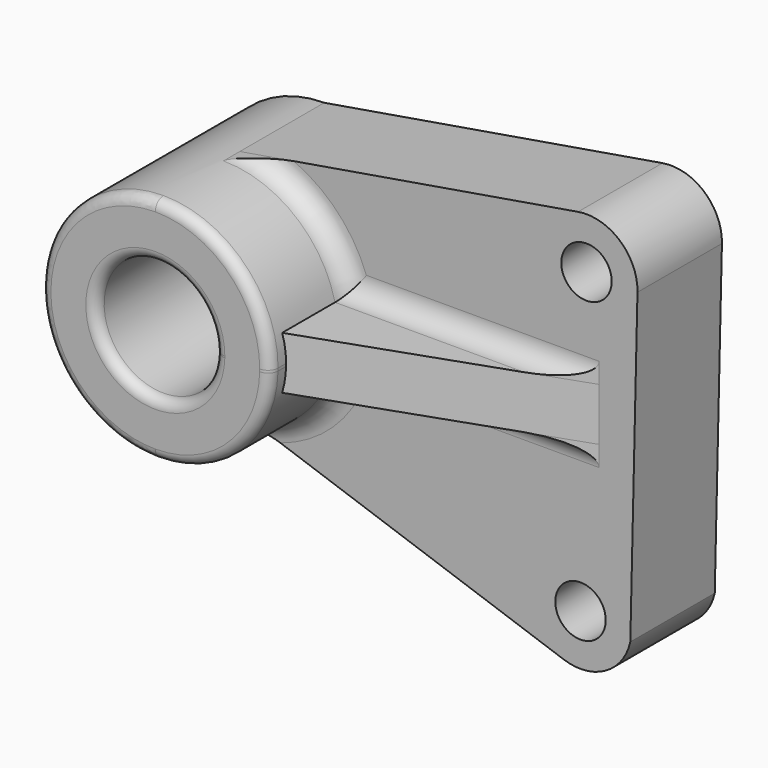
from build123d import *

# Parameters (mm, degrees)
F1_DEPTH     = 12.7
F2_DEPTH     = 25.4
F3_R         = 3.0339595682
F4_DEPTH     = 25.4
F5_R         = 1.2264204897
F7_DEPTH     = 3.175
F8_T4_ANGLE  = 97.0773840638
F8_T9_DEPTH  = 34.7132171162
F8_T14_ANGLE = 97.0773840638
F8_T19_DEPTH = 34.7132171162


# Not quite as in the source:
# - a fillet or chamfer that OpenCascade refuses, or shapes differently, is made with other operations: its cross-section is extruded or revolved along the edge and cut away or added


with BuildPart() as f1:
    # F0 (on Front) → F1 (new body)
    with BuildSketch(Plane.XZ):
        with BuildLine():
            ThreePointArc((0, -13.789825828), (9.6376295499, -9.8628288552), (13.7861481364, -0.3184586768))
            ThreePointArc((13.7861481364, -0.3184586768), (13.7889063745, -0.1592399559), (13.789825828, 0))
            ThreePointArc((13.789825828, 0), (9.7508793544, 9.7508793544), (0, 13.789825828))
            ThreePointArc((0, 13.789825828), (-13.789825828, 0), (0, -13.789825828))
        make_face()
        with BuildLine():
            ThreePointArc((7.1353728529, -0.1648264167), (-7.1368004494, 0.0824187037), (7.137276336, 0))
            ThreePointArc((7.137276336, 0), (7.1368004494, -0.0824187037), (7.1353728529, -0.1648264167))
        make_face(mode=Mode.SUBTRACT)
        with BuildLine():
            ThreePointArc((13.789825828, 0), (13.7889063745, -0.1592399559), (13.7861481364, -0.3184586768))
            ThreePointArc((13.7861481364, -0.3184586768), (9.6376295499, -9.8628288552), (0, -13.789825828))
            Line((0, -13.789825828), (38.9815755188, -27.3394305259))
            ThreePointArc((38.9815755188, -27.3394305259), (43.9885292005, -26.9000346666), (46.9867042389, -22.8659795937))
            Line((46.9867042389, -22.8659795937), (47.8485122544, 14.4418842975))
            ThreePointArc((47.8485122544, 14.4418842975), (45.7311207367, 19.22142423), (40.6978976177, 20.6335197794))
            Line((40.6978976177, 20.6335197794), (0, 13.789825828))
            ThreePointArc((0, 13.789825828), (9.7508793544, 9.7508793544), (13.789825828, 0))
        make_face()
    extrude(amount=F1_DEPTH)

    # F0 (on Front) → F2 (join)
    with BuildSketch(Plane.XZ):
        with BuildLine():
            ThreePointArc((0, -13.789825828), (9.6376295499, -9.8628288552), (13.7861481364, -0.3184586768))
            ThreePointArc((13.7861481364, -0.3184586768), (13.7889063745, -0.1592399559), (13.789825828, 0))
            ThreePointArc((13.789825828, 0), (9.7508793544, 9.7508793544), (0, 13.789825828))
            ThreePointArc((0, 13.789825828), (-13.789825828, 0), (0, -13.789825828))
        make_face()
        with BuildLine():
            ThreePointArc((7.1353728529, -0.1648264167), (-7.1368004494, 0.0824187037), (7.137276336, 0))
            ThreePointArc((7.137276336, 0), (7.1368004494, -0.0824187037), (7.1353728529, -0.1648264167))
        make_face(mode=Mode.SUBTRACT)
    extrude(amount=F2_DEPTH)

    # F3 (on face) → F4 (cut)
    with BuildSketch(Plane.XZ.offset(12.7)):
        with Locations((40.9957959094, -21.5446131849)):
            Circle(F3_R)
        with Locations((41.715248914, 14.5835620822)):
            Circle(F3_R)
    extrude(amount=-F4_DEPTH, mode=Mode.SUBTRACT)

    # F5
    f5_edges = [f1.edges().sort_by_distance(p)[0] for p in [
        (0, -25.4, 13.789826),
        (-7.137276, -25.4, 0),
    ]]
    fillet(f5_edges, radius=F5_R)

    # F6 (on Top) → F7 (join, symmetric)
    with BuildSketch(Plane.XY):
        Polygon((13.3344670758, -12.2673781589), (13.3344670758, -23.1246650219), (44.4674044847, -12.2673781589), align=None)
    extrude(amount=F7_DEPTH, both=True)

    # F8: fillet of radius 2.4528409794 on 4 edges, made by hand


with BuildPart() as f8_tool2:
    # F8_s3 → F8_t4 (revolve)
    with BuildSketch(Plane(origin=(0, 0, 0), x_dir=(0, 1, 0), z_dir=(0.0543746304, 0, 0.9985206055))):
        with BuildLine():
            ThreePointArc((-15.1528409794, -13.789825828), (-13.4184204897, -14.5082463177), (-12.7, -16.2426668074))
            Line((-12.7, -16.2426668074), (-12.6509431804, -16.2426668074))
            Line((-12.6509431804, -16.2426668074), (-12.6509431804, -13.7407690084))
            Line((-12.6509431804, -13.7407690084), (-15.1528409794, -13.7407690084))
            Line((-15.1528409794, -13.7407690084), (-15.1528409794, -13.789825828))
        make_face()
    revolve(axis=Axis((0, -12.7, 0), (0, 1, 0)), revolution_arc=F8_T4_ANGLE)

    split(bisect_by=Plane(origin=(-4.2765210661, 0, -12.3033499954), x_dir=(0, 1, 0), z_dir=(0.3283216608, 0, 0.9445659781)), keep=Keep.TOP)


with BuildPart() as f1_1:
    add(f1.part)

    # F8_t1: union F8_tool2
    add(f8_tool2.part)


with BuildPart() as f8_tool7:
    # F8_s8 → F8_t9 (new body)
    with BuildSketch(Plane.YZ.offset(45.6797155903)):
        with BuildLine():
            ThreePointArc((-12.7, -5.6278409794), (-13.4184204897, -3.8934204897), (-15.1528409794, -3.175))
            Line((-15.1528409794, -3.175), (-15.1528409794, -3.1259431804))
            Line((-15.1528409794, -3.1259431804), (-12.6509431804, -3.1259431804))
            Line((-12.6509431804, -3.1259431804), (-12.6509431804, -5.6278409794))
            Line((-12.6509431804, -5.6278409794), (-12.7, -5.6278409794))
        make_face()
    extrude(amount=-F8_T9_DEPTH)

    split(bisect_by=Plane(origin=(8.6359194604, -24.7632344453, 0), x_dir=(0, 0, 1), z_dir=(-0.3292899537, 0.9442288528, 0)), keep=Keep.TOP)


with BuildPart() as f1_2:
    add(f1_1.part)

    # F8_t6: union F8_tool7
    add(f8_tool7.part)


with BuildPart() as f8_tool12:
    # F8_s13 → F8_t14 (revolve)
    with BuildSketch(Plane(origin=(0, 0, 0), x_dir=(0, 1, 0), z_dir=(-0.9842130406, 0, -0.1769878264))):
        with BuildLine():
            ThreePointArc((-15.1528409794, -13.789825828), (-13.4184204897, -14.5082463177), (-12.7, -16.2426668074))
            Line((-12.7, -16.2426668074), (-12.6509431804, -16.2426668074))
            Line((-12.6509431804, -16.2426668074), (-12.6509431804, -13.7407690084))
            Line((-12.6509431804, -13.7407690084), (-15.1528409794, -13.7407690084))
            Line((-15.1528409794, -13.7407690084), (-15.1528409794, -13.789825828))
        make_face()
    revolve(axis=Axis((0, -12.7, 0), (0, 1, 0)), revolution_arc=F8_T14_ANGLE)

    split(bisect_by=Plane(origin=(-2.2551070217, 0, 13.4106106059), x_dir=(0, 1, 0), z_dir=(0.1658301489, 0, -0.9861543296)), keep=Keep.TOP)


with BuildPart() as f1_3:
    add(f1_2.part)

    # F8_t11: union F8_tool12
    add(f8_tool12.part)


with BuildPart() as f8_tool17:
    # F8_s18 → F8_t19 (new body)
    with BuildSketch(Plane.YZ.offset(45.6797155903)):
        with BuildLine():
            ThreePointArc((-12.7, 5.6278409794), (-13.4184204897, 3.8934204897), (-15.1528409794, 3.175))
            Line((-15.1528409794, 3.175), (-15.1528409794, 3.1259431804))
            Line((-15.1528409794, 3.1259431804), (-12.6509431804, 3.1259431804))
            Line((-12.6509431804, 3.1259431804), (-12.6509431804, 5.6278409794))
            Line((-12.6509431804, 5.6278409794), (-12.7, 5.6278409794))
        make_face()
    extrude(amount=-F8_T19_DEPTH)

    split(bisect_by=Plane(origin=(8.6359194604, -24.7632344453, 0), x_dir=(0, 0, 1), z_dir=(-0.3292899537, 0.9442288528, 0)), keep=Keep.TOP)


with BuildPart() as f1_4:
    add(f1_3.part)

    # F8_t16: union F8_tool17
    add(f8_tool17.part)


solid = f1_4.part
